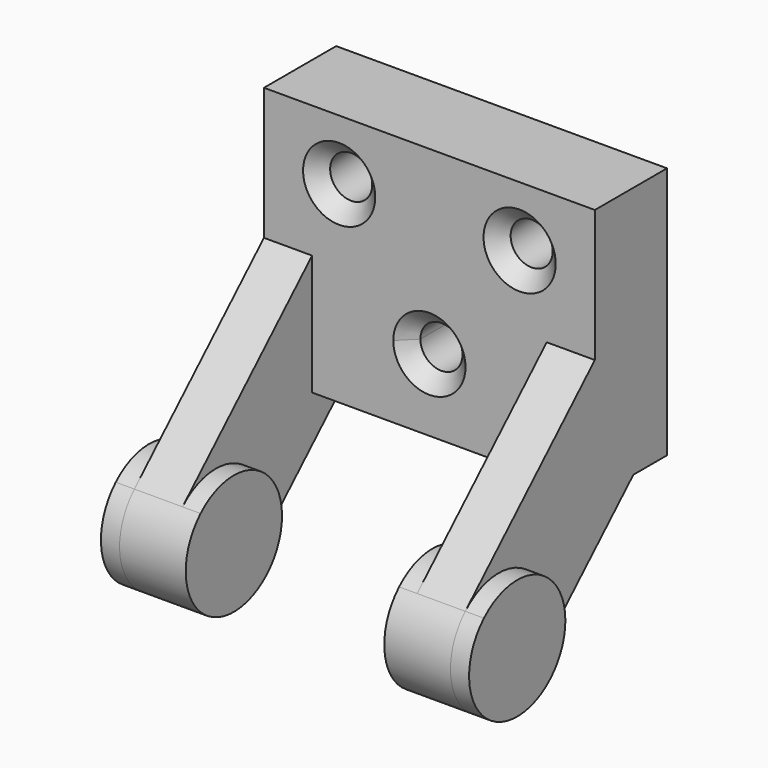
from build123d import *

# Parameters (mm, degrees)
F0_W           = 55
F0_H           = 42
F1_DEPTH       = 15
F3_DEPTH       = 8
F4_DEPTH       = 3.1
F4_DEPTH_BACK  = 11
F6_D           = 7
F6_CSINK_D     = 12
F6_CSINK_ANGLE = 90


# Not quite as in the source:
# - a pattern or mirror of a feature is missing from the dataset's text; its kind, count and spacing are read off the source's solid


with BuildPart() as f1:
    # F0 (on Front) → F1 (new body)
    with BuildSketch(Plane.XZ):
        with Locations((0, -21)):
            Rectangle(F0_W, F0_H)
    extrude(amount=-F1_DEPTH)

    # F2 (on face) → F3 (join)
    with BuildSketch(Plane.YZ.offset(27.5)):
        with BuildLine():
            Line((0, -42), (0, -21.960586854))
            Line((0, -21.960586854), (-26.9221419573, -47.7830788612))
            ThreePointArc((-26.9221419573, -47.7830788612), (-16.0770814164, -45.8015919972), (-10, -55))
            ThreePointArc((-10, -55), (-10.8015919972, -58.9229185836), (-13.0778580427, -62.2169211388))
            Line((-13.0778580427, -62.2169211388), (8, -42))
            Line((8, -42), (0, -42))
        make_face()
        with BuildLine():
            ThreePointArc((-10, -55), (-16.0770814164, -45.8015919972), (-26.9221419573, -47.7830788612))
            Line((-26.9221419573, -47.7830788612), (-13.0778580427, -62.2169211388))
            ThreePointArc((-13.0778580427, -62.2169211388), (-10.8015919972, -58.9229185836), (-10, -55))
        make_face()
    f3 = extrude(amount=-F3_DEPTH)

    # F3_copies: F3 across plane
    add(f3.mirror(Plane(origin=(0, 0, 0), x_dir=(0, 0, -1), z_dir=(-1, 0, 0))))

    # F2 (on face) → F4 (join, two sides)
    with BuildSketch(Plane.YZ.offset(27.5)) as f4_sk:
        with BuildLine():
            Line((-13.0778580427, -62.2169211388), (-26.9221419573, -47.7830788612))
            ThreePointArc((-26.9221419573, -47.7830788612), (-27.2169211388, -61.9221419573), (-13.0778580427, -62.2169211388))
        make_face()
        with BuildLine():
            ThreePointArc((-10, -55), (-16.0770814164, -45.8015919972), (-26.9221419573, -47.7830788612))
            Line((-26.9221419573, -47.7830788612), (-13.0778580427, -62.2169211388))
            ThreePointArc((-13.0778580427, -62.2169211388), (-10.8015919972, -58.9229185836), (-10, -55))
        make_face()
    f4 = extrude(amount=F4_DEPTH) + extrude(f4_sk.sketch, amount=-F4_DEPTH_BACK)

    # F4_copies: F4 across plane
    add(f4.mirror(Plane(origin=(0, 0, 0), x_dir=(0, 0, -1), z_dir=(-1, 0, 0))))

    # F6 (through all)
    with Locations(Plane.XZ):
        with Locations((-15, -10), (0, -30)):
            f6 = CounterSinkHole(F6_D / 2, F6_CSINK_D / 2, counter_sink_angle=F6_CSINK_ANGLE)

    # F6_copies: F6 across plane
    add(f6.mirror(Plane(origin=(0, 0, 0), x_dir=(0, 0, 1), z_dir=(1, 0, 0))), mode=Mode.SUBTRACT)


solid = f1.part
